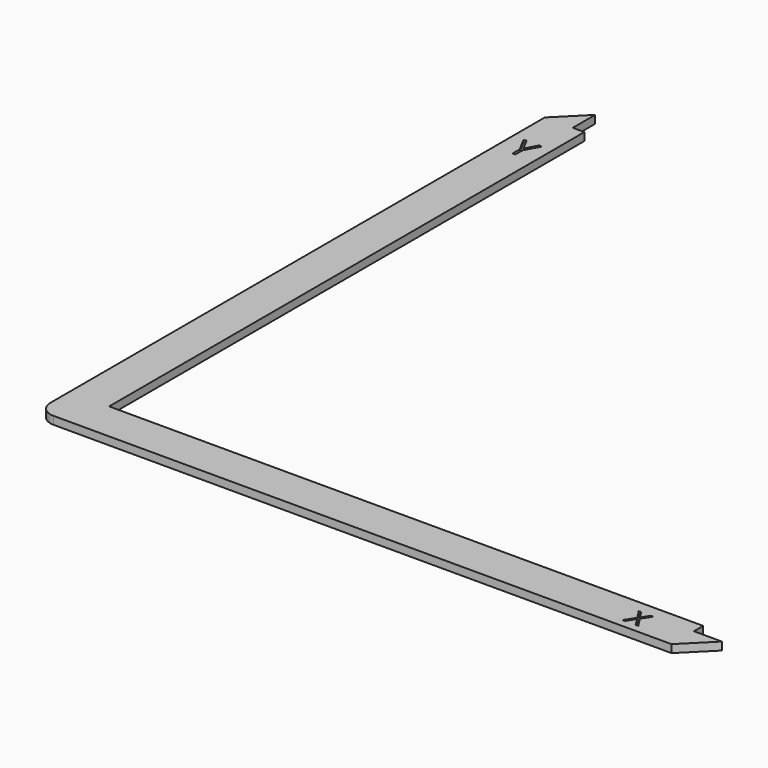
from build123d import *

# Parameters (mm, degrees)
F1_DEPTH       = 1
F3_DEPTH       = 1
F4_TEXT_SIZE   = 4.1666666667
F4_TEXT_SIZE_2 = 3.4722222222
F5_DEPTH       = 0.3
F6_R           = 0.1
F7_R           = 2


# Not quite as in the source:
# - Text() gives the source's letters only with a copy of the font that has no kerning and outlines rounded to 1/6400 em; it was checked with that copy


with BuildPart() as f1:
    # F0 (on Top) → F1 (new body)
    with BuildSketch(Plane.XY):
        Polygon((0, 5), (0, 0), (5, 0), (80, 0), (80, 5), (5, 5), (5, 80), (0, 80), align=None)
    extrude(amount=F1_DEPTH)

    # F2 (on face) → F3 (join, through all)
    with BuildSketch(Plane.XY.offset(1)):
        Polygon((3.5355339059, 83.5355339059), (0, 80), (3.5355339059, 80), align=None)
        Polygon((80, 3.5355339059), (80, 0), (83.5355339059, 3.5355339059), align=None)
    extrude(amount=-F3_DEPTH)

    # F4 (on face) → F5 (cut)
    with BuildSketch(Plane.XY.offset(1)):
        with Locations((1.3333333333, 72)):
            Text('Y', F4_TEXT_SIZE, font='Open Sans', text_align=(TextAlign.LEFT, TextAlign.BOTTOM))
        with Locations((73.0094401042, 1)):
            Text('X', F4_TEXT_SIZE_2, font='Open Sans', text_align=(TextAlign.LEFT, TextAlign.BOTTOM))
    extrude(amount=-F5_DEPTH, mode=Mode.SUBTRACT)

    # F6
    f6_edges = [f1.edges().sort_by_distance(p)[0] for p in [
        (80, 4.267767, 0),
    ]]
    fillet(f6_edges, radius=F6_R)

    # F7
    f7_edges = [f1.edges().sort_by_distance(p)[0] for p in [
        (0, 0, 0.5),
    ]]
    fillet(f7_edges, radius=F7_R)


solid = f1.part
